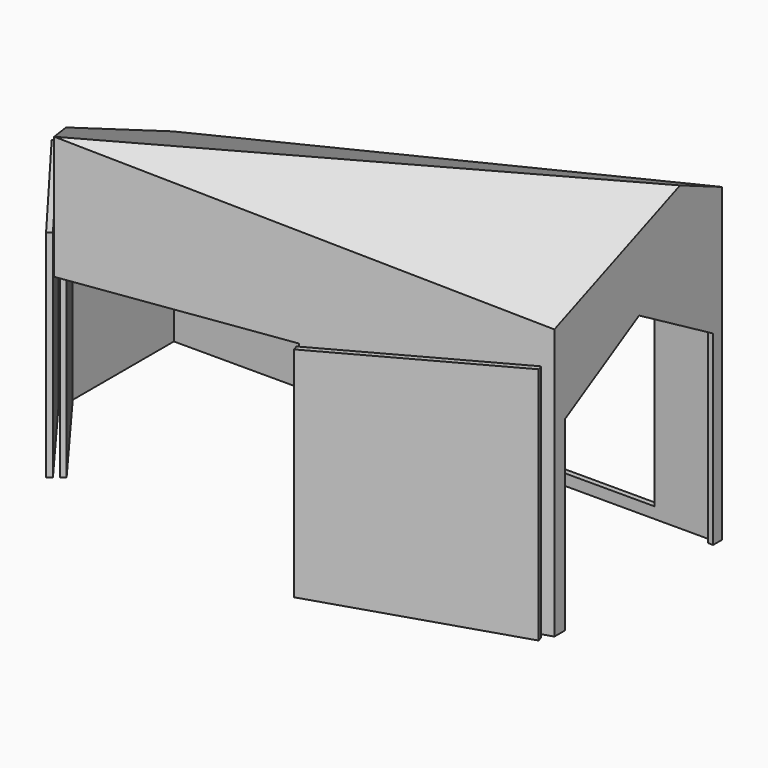
from build123d import *

# Parameters (mm, degrees)
F1_DEPTH  = 86.106
F6_W      = 240.2444779873
F6_H      = 147.931613028
F7_DEPTH  = 60.706
F10_W     = 135.2960467339
F10_H     = 94.6298297495
F11_DEPTH = 41.148
F13_T     = -1.27
F14_DEPTH = 2.54
F16_DEPTH = 2.54
F18_DEPTH = 2.54
F19_W     = 30.9821236879
F19_H     = 45.3865022864
F19_W_2   = 32.3204575107
F20_DEPTH = 2.54
F23_START = 1.27
F23_DEPTH = 1.27
F25_START = 1.27
F25_DEPTH = 1.27


# Not quite as in the source:
# - the program builds the solid bodies; features that only make, move or delete a surface that nothing else refers to are left out


with BuildPart() as f1:
    # F0 (on Top) → F1 (new body)
    with BuildSketch(Plane.XY):
        Polygon((63.8810023665, 46.616720651), (-66.6749998927, 46.616720651), (-66.6749998927, 14.8563552648), (-30.8609995991, -33.4036462009), (63.8810023665, -3.1776451506), align=None)
    extrude(amount=F1_DEPTH)

    # F6 (on 3pt) + F3 (on face) → F7 (cut)
    with BuildSketch(Plane(origin=(-14.9985821509, 27.4688705788, 63.5316546184), x_dir=(0.9773177277, 0.084046153, 0.1943869934), z_dir=(-0.2117783252, 0.387857422, 0.897059954))):
        with Locations((-7.4320882559, 3.8242153823)):
            Rectangle(F6_W, F6_H)
    with BuildSketch(Plane(origin=(0, 46.616720651, 0), x_dir=(-1, 0, 0), z_dir=(0, 1, 0))):
        Polygon((-63.8810023665, 86.106), (-63.8810023665, 62.2684090482), (-14.7184757516, 62.2684090482), (66.6749998927, 62.2684090482), (66.6749998927, 86.106), align=None)
    extrude(amount=F7_DEPTH, dir=(-0.2117783252, 0.387857422, 0.897059954), mode=Mode.SUBTRACT)

    # F10 (on 3pt) → F11 (cut)
    with BuildSketch(Plane(origin=(24.5709511473, -27.5043865165, 68.6225243158), x_dir=(0.9489607702, 0.1173380711, -0.2927545622), z_dir=(0.315394129, -0.3530478726, 0.8808426324))):
        with Locations((4.6633481979, 24.4434149936)):
            Rectangle(F10_W, F10_H)
    extrude(amount=F11_DEPTH, mode=Mode.SUBTRACT)

    # F13
    f13_openings = [f1.faces().sort_by_distance(p)[0] for p in [
        (-1.661142, 14.401339, 0),
    ]]
    offset(amount=F13_T, openings=f13_openings)

    # F12 (on face) → F14 (cut)
    with BuildSketch(Plane(origin=(-35.8865647103, -26.6316079577, 0), x_dir=(0.5959348457, -0.8030327886, 0), z_dir=(-0.8030327886, -0.5959348457, 0))):
        Polygon((-19.9140961726, 51.251806932), (-19.9140961726, 0), (8.4330781245, 0), (8.4330781245, 56.7850737445), align=None)
    extrude(amount=-F14_DEPTH, mode=Mode.SUBTRACT)

    # F15 (on face) → F16 (cut)
    with BuildSketch(Plane(origin=(6.8214823825, -21.38162095, 0), x_dir=(0.9526906855, 0.3039415366, 0), z_dir=(0.3039415366, -0.9526906855, 0))):
        Polygon((9.0930175873, 51.884541691), (-39.55374242, 56.7850737445), (-39.55374242, 0), (9.0930175873, 0), align=None)
    extrude(amount=-F16_DEPTH, mode=Mode.SUBTRACT)

    # F17 (on face) → F18 (cut)
    with BuildSketch(Plane.YZ.offset(63.8810023665)):
        Polygon((0, 44.2713387311), (0, 0), (43.9940905122, 0), (43.9940905122, 44.2713387311), (21.9970452561, 56.9713387311), align=None)
    extrude(amount=-F18_DEPTH, mode=Mode.SUBTRACT)

    # F19 (on face) → F20 (cut)
    with BuildSketch(Plane(origin=(0, 46.616720651, 0), x_dir=(-1, 0, 0), z_dir=(0, 1, 0))):
        with Locations((-33.4093561396, 25.3466918366)):
            Rectangle(F19_W, F19_H)
        with Locations((4.2059472762, 25.3466918366)):
            Rectangle(F19_W_2, F19_H)
    extrude(amount=-F20_DEPTH, mode=Mode.SUBTRACT)


with BuildPart() as f23:
    # F22 (on face) → F23 (new body)
    with BuildSketch(Plane(origin=(6.8214823825, -21.38162095, 0), x_dir=(0.9526906855, 0.3039415366, 0), z_dir=(0.3039415366, -0.9526906855, 0)).offset(F23_START)):
        Polygon((57.7399830757, 56.7830335389), (9.0930175873, 51.884541691), (9.0930175873, 0), (57.7399830757, 0), align=None)
    extrude(amount=F23_DEPTH)


with BuildPart() as f25:
    # F24 (on face) → F25 (new body)
    with BuildSketch(Plane(origin=(-35.8865647103, -26.6316079577, 0), x_dir=(0.5959348457, -0.8030327886, 0), z_dir=(-0.8030327886, -0.5959348457, 0)).offset(F25_START)):
        Polygon((-19.9140961726, 0), (-19.9140961726, 51.251806932), (-48.4388518792, 55.7814475499), (-48.4388518792, 0), align=None)
    extrude(amount=F25_DEPTH)


solid = Compound([f1.part, f23.part, f25.part])
